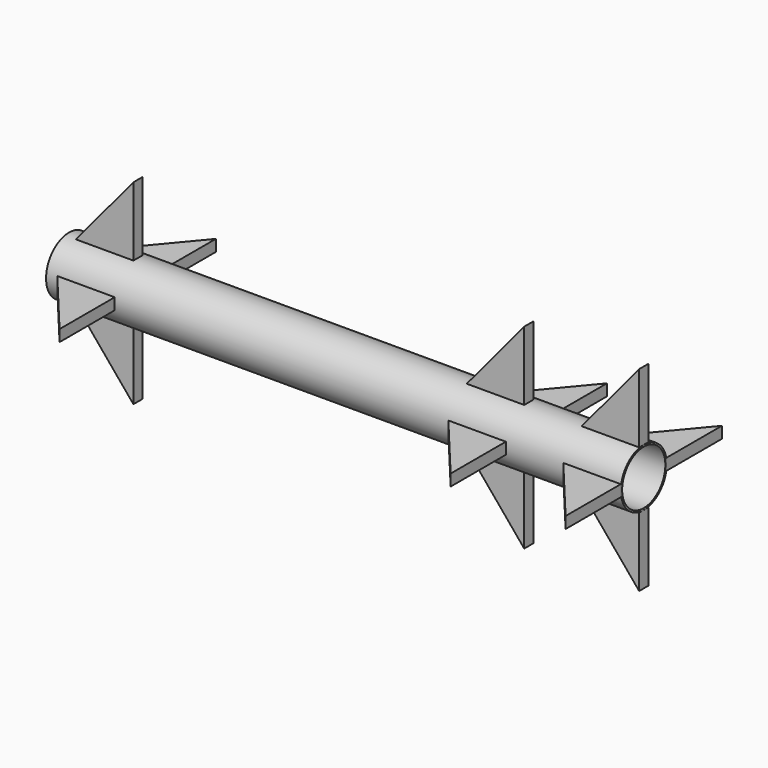
from build123d import *

# Parameters (mm, degrees)
F1_R          = 76.2
F2_DEPTH      = 762
F2_DEPTH_BACK = 762
F4_DEPTH      = 15.24
F4_DEPTH_BACK = 15.24
F6_DEPTH      = 15.24
F6_DEPTH_BACK = 15.24
F7_T          = -4.572


# Not quite as in the source:
# - the program builds the solid bodies; features that only make, move or delete a surface that nothing else refers to are left out


with BuildPart() as f2:
    # F1 (on Right) → F2 (new body, two sides)
    with BuildSketch(Plane.YZ) as f2_sk:
        Circle(F1_R)
    extrude(amount=F2_DEPTH)
    extrude(f2_sk.sketch, amount=-F2_DEPTH_BACK)

    # F7
    f7_openings = [f2.faces().sort_by_distance(p)[0] for p in [
        (762, 0, 0),
    ]]
    offset(amount=F7_T, openings=f7_openings)


with BuildPart() as f4:
    # F0 (on Top) → F4 (new body, two sides)
    with BuildSketch(Plane.XY) as f4_sk:
        Polygon((-732.2247028351, 76.2), (-579.8247028351, 76.2), (-579.8247028351, 259.08), align=None)
    extrude(amount=F4_DEPTH)
    extrude(f4_sk.sketch, amount=-F4_DEPTH_BACK)


with BuildPart() as f4b:
    # F0 (on Top) → F4, piece 2 (new body, two sides)
    with BuildSketch(Plane.XY) as f4_2_sk:
        Polygon((-579.8247028351, -259.08), (-579.8247028351, -76.2), (-732.2247028351, -76.2), align=None)
    extrude(amount=F4_DEPTH)
    extrude(f4_2_sk.sketch, amount=-F4_DEPTH_BACK)


with BuildPart() as f4c:
    # F0 (on Top) → F4, piece 3 (new body, two sides)
    with BuildSketch(Plane.XY) as f4_3_sk:
        Polygon((457.2, -259.08), (457.2, -76.2), (304.8, -76.2), align=None)
    extrude(amount=F4_DEPTH)
    extrude(f4_3_sk.sketch, amount=-F4_DEPTH_BACK)


with BuildPart() as f4d:
    # F0 (on Top) → F4, piece 4 (new body, two sides)
    with BuildSketch(Plane.XY) as f4_4_sk:
        Polygon((304.8, 76.2), (457.2, 76.2), (457.2, 259.08), align=None)
    extrude(amount=F4_DEPTH)
    extrude(f4_4_sk.sketch, amount=-F4_DEPTH_BACK)


with BuildPart() as f4e:
    # F0 (on Top) → F4, piece 5 (new body, two sides)
    with BuildSketch(Plane.XY) as f4_5_sk:
        Polygon((609.6, 76.2), (762, 76.2), (762, 259.08), align=None)
    extrude(amount=F4_DEPTH)
    extrude(f4_5_sk.sketch, amount=-F4_DEPTH_BACK)


with BuildPart() as f4f:
    # F0 (on Top) → F4, piece 6 (new body, two sides)
    with BuildSketch(Plane.XY) as f4_6_sk:
        Polygon((762, -259.08), (762, -76.2), (609.6, -76.2), align=None)
    extrude(amount=F4_DEPTH)
    extrude(f4_6_sk.sketch, amount=-F4_DEPTH_BACK)


with BuildPart() as f6:
    # F5 (on Front) → F6 (new body, two sides)
    with BuildSketch(Plane.XZ) as f6_sk:
        Polygon((762, -76.2), (609.6, -76.2), (762, -259.08), align=None)
    extrude(amount=F6_DEPTH)
    extrude(f6_sk.sketch, amount=-F6_DEPTH_BACK)


with BuildPart() as f6b:
    # F5 (on Front) → F6, piece 2 (new body, two sides)
    with BuildSketch(Plane.XZ) as f6_2_sk:
        Polygon((762, 259.08), (609.6, 76.2), (762, 76.2), align=None)
    extrude(amount=F6_DEPTH)
    extrude(f6_2_sk.sketch, amount=-F6_DEPTH_BACK)


with BuildPart() as f6c:
    # F5 (on Front) → F6, piece 3 (new body, two sides)
    with BuildSketch(Plane.XZ) as f6_3_sk:
        Polygon((457.2, -76.2), (304.8, -76.2), (457.2, -259.08), align=None)
    extrude(amount=F6_DEPTH)
    extrude(f6_3_sk.sketch, amount=-F6_DEPTH_BACK)


with BuildPart() as f6d:
    # F5 (on Front) → F6, piece 4 (new body, two sides)
    with BuildSketch(Plane.XZ) as f6_4_sk:
        Polygon((457.2, 259.08), (304.8, 76.2), (457.2, 76.2), align=None)
    extrude(amount=F6_DEPTH)
    extrude(f6_4_sk.sketch, amount=-F6_DEPTH_BACK)


with BuildPart() as f6e:
    # F5 (on Front) → F6, piece 5 (new body, two sides)
    with BuildSketch(Plane.XZ) as f6_5_sk:
        Polygon((-731.52, 76.2), (-579.12, 76.2), (-579.12, 259.08), align=None)
    extrude(amount=F6_DEPTH)
    extrude(f6_5_sk.sketch, amount=-F6_DEPTH_BACK)


with BuildPart() as f6f:
    # F5 (on Front) → F6, piece 6 (new body, two sides)
    with BuildSketch(Plane.XZ) as f6_6_sk:
        Polygon((-579.12, -259.08), (-579.12, -76.2), (-731.52, -76.2), align=None)
    extrude(amount=F6_DEPTH)
    extrude(f6_6_sk.sketch, amount=-F6_DEPTH_BACK)


solid = Compound([f2.part, f4.part, f4b.part, f4c.part, f4d.part, f4e.part, f4f.part, f6.part, f6b.part, f6c.part, f6d.part, f6e.part, f6f.part])
